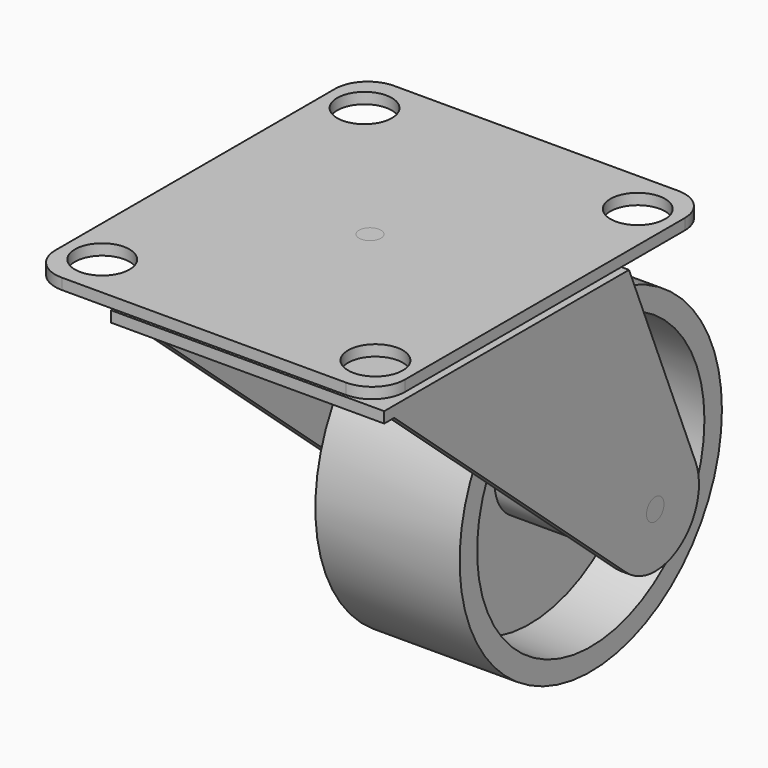
from build123d import *

# Parameters (mm, degrees)
F0_R      = 13
F0_R_2    = 4
F1_DEPTH  = 1
F0_R_3    = 15
F0_R_4    = 1
F2_DEPTH  = 6.6
F4_W      = 25
F4_H      = 28
F4_R      = 1
F5_DEPTH  = 0.5
F7_R      = 1
F8_DEPTH  = 1
F11_R     = 2.5
F11_R_2   = 1
F12_DEPTH = 1
F13_R     = 1
F14_DEPTH = 1
F13_R_2   = 2.5
F15_DEPTH = 3.5
F16_R     = 1
F17_DEPTH = 1
F18_R     = 1
F19_DEPTH = 12.5


with BuildPart() as f1:
    # F0 (on Right) → F1 (new body, symmetric)
    with BuildSketch(Plane.YZ):
        Circle(F0_R)
        Circle(F0_R_2, mode=Mode.SUBTRACT)
    extrude(amount=F1_DEPTH, both=True)

    # F0 (on Right) → F2 (join, symmetric)
    with BuildSketch(Plane.YZ):
        Circle(F0_R_3)
        Circle(F0_R, mode=Mode.SUBTRACT)
        Circle(F0_R_2)
        Circle(F0_R_4, mode=Mode.SUBTRACT)
    extrude(amount=F2_DEPTH, both=True)


with BuildPart() as f5:
    # F4 (on offset) → F5 (new body, symmetric)
    with BuildSketch(Plane.XY.offset(20)):
        with Locations((0, -17)):
            Rectangle(F4_W, F4_H)
        with Locations((0, -17)):
            Circle(F4_R, mode=Mode.SUBTRACT)
    extrude(amount=F5_DEPTH, both=True)

    # F7 (on offset) → F8 (join)
    with BuildSketch(Plane.YZ.offset(11.5)):
        with BuildLine():
            Line((-3, 20.5), (-31, 20.5))
            Line((-31, 20.5), (-3.2939715582, -3.7616155271))
            ThreePointArc((-3.2939715582, -3.7616155271), (2.9064564522, -4.0684777118), (4.6263525904, 1.8965394035))
            Line((4.6263525904, 1.8965394035), (-3, 20.5))
        make_face()
        Circle(F7_R, mode=Mode.SUBTRACT)
    extrude(amount=F8_DEPTH)

    # F9: F5 across plane


with BuildPart() as f5_1:
    add(f5.part)
    add(f5.part.mirror(Plane.YZ))


with BuildPart() as f12:
    # F11 (on offset) → F12 (new body)
    with BuildSketch(Plane.XY.offset(25)):
        with BuildLine():
            ThreePointArc((-16, -33), (-15.1213203436, -35.1213203436), (-13, -36))
            Line((-13, -36), (13, -36))
            ThreePointArc((13, -36), (15.1213203436, -35.1213203436), (16, -33))
            Line((16, -33), (16, -1))
            ThreePointArc((16, -1), (15.1213203436, 1.1213203436), (13, 2))
            Line((13, 2), (-13, 2))
            ThreePointArc((-13, 2), (-15.1213203436, 1.1213203436), (-16, -1))
            Line((-16, -1), (-16, -33))
        make_face()
        with Locations((-12.5, -32)):
            Circle(F11_R, mode=Mode.SUBTRACT)
        with Locations((12.5, -32)):
            Circle(F11_R, mode=Mode.SUBTRACT)
        with Locations((-12.5, -2)):
            Circle(F11_R, mode=Mode.SUBTRACT)
        with Locations((0, -17)):
            Circle(F11_R_2, mode=Mode.SUBTRACT)
        with Locations((12.5, -2)):
            Circle(F11_R, mode=Mode.SUBTRACT)
    extrude(amount=-F12_DEPTH)


with BuildPart() as f14:
    # F13 (on face) → F14 (new body, symmetric)
    with BuildSketch(Plane.XY.offset(20.5)):
        with Locations((0, -17)):
            Circle(F13_R)
    extrude(amount=F14_DEPTH, both=True)

    # F13 (on face) → F15 (join)
    with BuildSketch(Plane.XY.offset(20.5)):
        with Locations((0, -17)):
            Circle(F13_R_2)
        with Locations((0, -17)):
            Circle(F13_R, mode=Mode.SUBTRACT)
    extrude(amount=F15_DEPTH)

    # F16 (on face) → F17 (join, symmetric)
    with BuildSketch(Plane.XY.offset(24)):
        with Locations((0, -17)):
            Circle(F16_R)
    extrude(amount=F17_DEPTH, both=True)


with BuildPart() as f19:
    # F18 (on Right) → F19 (new body, symmetric)
    with BuildSketch(Plane.YZ):
        Circle(F18_R)
    extrude(amount=F19_DEPTH, both=True)


solid = Compound([f1.part, f5_1.part, f12.part, f14.part, f19.part])
